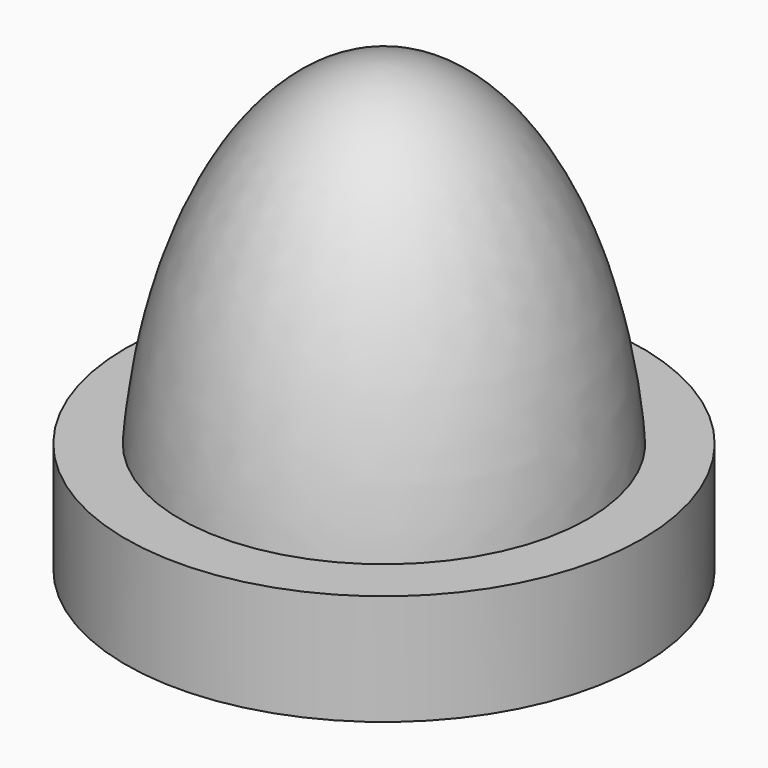
from build123d import *

# Parameters (mm, degrees)
F2_R     = 3
F3_DEPTH = 10.16


# Not quite as in the source:
# - a feature names something its author has since deleted; it is built from what else it names


with BuildPart() as f1:
    # F0 (on Front) → F1 (revolve)
    with BuildSketch(Plane.XZ):
        with BuildLine():
            Line((-5.9580963571, 0), (-7.5407535769, 0))
            Line((-7.5407535769, 0), (-7.5407535769, -3.2317098148))
            Line((-7.5407535769, -3.2317098148), (-5.9580963571, -3.2317098148))
            add(Edge.make_bspline(
                [(-5.9580963571, 0), (-6.0799979609, -1.6158549074), (-5.9580963571, -3.2317098148)],
                knots=[1.4287221918, 1.4287221918, 1.4287221918, 1.7128704618, 1.7128704618, 1.7128704618], degree=2, weights=[1, 0.9899244352, 1]))
        make_face()
        with BuildLine():
            add(Edge.make_bspline(
                [(0, 9.7958194092), (-5.2190905892, 9.7958194092), (-5.9580963571, 0)],
                knots=[0, 0, 0, 1.4287221918, 1.4287221918, 1.4287221918], degree=2, weights=[1, 0.7555119637, 1]))
            add(Edge.make_bspline(
                [(-5.9580963571, 0), (-6.0799979609, -1.6158549074), (-5.9580963571, -3.2317098148)],
                knots=[1.4287221918, 1.4287221918, 1.4287221918, 1.7128704618, 1.7128704618, 1.7128704618], degree=2, weights=[1, 0.9899244352, 1]))
            Line((-5.9580963571, -3.2317098148), (0, -3.2317098148))
            Line((0, -3.2317098148), (0, 9.7958194092))
        make_face()
    revolve(axis=Axis((0, 0, 6.5636849072), (0, 0, -1)))

    # F2 (on face) → F3 (cut)
    with BuildSketch(Plane(origin=(0, 0, -3.2317098148), x_dir=(1, 0, 0), z_dir=(0, 0, -1))):
        Circle(F2_R)
    extrude(amount=-F3_DEPTH, mode=Mode.SUBTRACT)


solid = f1.part
